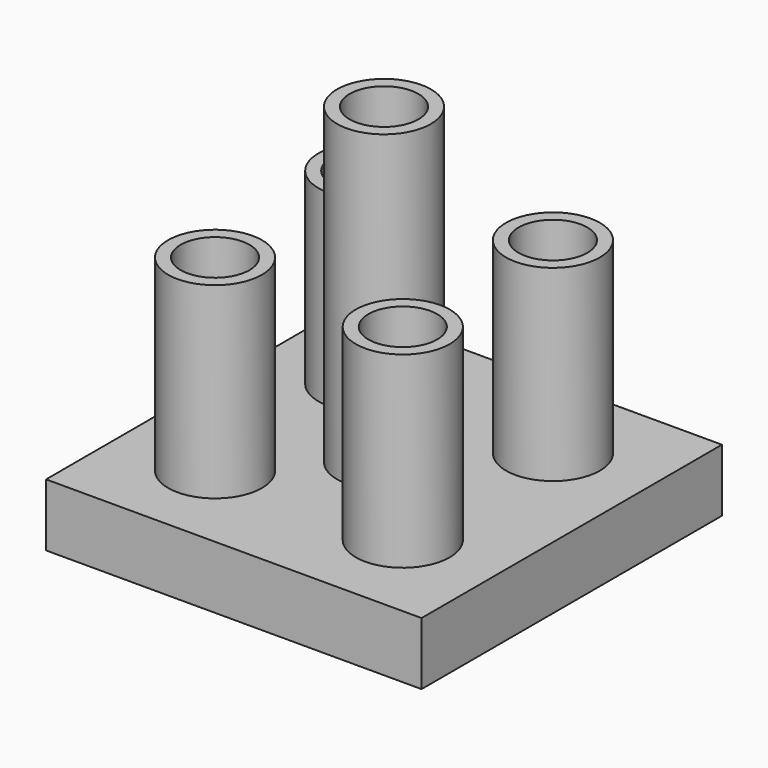
from build123d import *

# Parameters (mm, degrees)
F1_DEPTH    = 12.7
F2_R        = 9.525
F3_DEPTH    = 38.1
F4_T        = -2.54
F5_R        = 9.525
F6_DEPTH    = 63.5
F7_T        = 2.54
F7_T3_DEPTH = 12.7
F7_T5_DEPTH = 76.2
F7_T7_DEPTH = 76.2


# Not quite as in the source:
# - a shell that OpenCascade refuses in one call is made with other operations: the cavity is built on its own and cut out


with BuildPart() as f1:
    # F0 (on Top) → F1 (new body)
    with BuildSketch(Plane.XY):
        Polygon((-18.9360706136, 32.5840498031), (-57.0360706136, 32.5840498031), (-57.0360706136, -5.5159501969), (-57.0360706136, -43.6159501969), (-18.9360706136, -43.6159501969), (19.1639293864, -43.6159501969), (19.1639293864, -5.5159501969), (19.1639293864, 32.5840498031), align=None)
    extrude(amount=F1_DEPTH)

    # F2 (on face) → F3 (join)
    with BuildSketch(Plane.XY.offset(12.7)):
        with Locations((-37.9860706136, 13.5340498031)):
            Circle(F2_R)
        with Locations((0.1139293864, 13.5340498031)):
            Circle(F2_R)
        with Locations((-37.9860706136, -24.5659501969)):
            Circle(F2_R)
        with Locations((0.1139293864, -24.5659501969)):
            Circle(F2_R)
    extrude(amount=F3_DEPTH)

    # F4
    f4_openings = [f1.faces().sort_by_distance(p)[0] for p in [
        (0.113929, 13.53405, 50.8),
        (0.113929, -24.56595, 50.8),
        (-37.986071, -24.56595, 50.8),
        (-37.986071, 13.53405, 50.8),
    ]]
    offset(amount=F4_T, openings=f4_openings, kind=Kind.INTERSECTION)

    # F5 (on face) → F6 (join)
    with BuildSketch(Plane.XY.offset(12.7)):
        with Locations((-18.9360706136, -5.5159501969)):
            Circle(F5_R)
    extrude(amount=F6_DEPTH)

    # F7: shell of thickness 2.54, made by hand


with BuildPart() as f7_core1:
    # F7_t2: copy of F1
    add(f1.part)

    # the walls: a layer under each face that stays
    f7_faces = [f7_core1.faces().sort_by_distance(p)[0] for p in [
        (-18.9360706136, 30.0440498031, 6.35),
        (16.6239293864, -5.5159501969, 6.35),
        (-18.9360706136, -5.5159501969, 10.16),
        (-54.4960706136, -5.5159501969, 6.35),
        (-18.9360706136, -5.5159501969, 2.54),
        (-18.9360706136, -41.0759501969, 6.35),
        (-44.9710706136, 13.5340498031, 30.48),
        (-44.9710706136, -24.5659501969, 30.48),
        (-6.8710706136, 13.5340498031, 30.48),
        (-6.8710706136, -24.5659501969, 30.48),
        (-44.3360706136, 7.1840498031, 50.8),
        (-44.3360706136, -30.9159501969, 50.8),
        (-6.2360706136, 7.1840498031, 50.8),
        (-6.2360706136, -30.9159501969, 50.8),
        (-47.5110706136, 13.5340498031, 31.75),
        (-47.5110706136, -24.5659501969, 31.75),
        (-9.4110706136, 13.5340498031, 31.75),
        (-9.4110706136, -24.5659501969, 31.75),
        (-44.3360706136, -5.5159501969, 12.7),
        (-18.9360706136, 32.5840498031, 6.35),
        (-57.0360706136, -5.5159501969, 6.35),
        (19.1639293864, -5.5159501969, 6.35),
        (-18.9360706136, -43.6159501969, 6.35),
        (-28.4610706136, -5.5159501969, 44.45),
        (-18.9360706136, -5.5159501969, 0),
    ]]
    thicken(f7_faces, amount=-F7_T, mode=Mode.SUBTRACT)

    # F7_s4 → F7_t3 (cut)
    with BuildSketch(Plane.XY):
        Polygon((16.5985293864, 30.0186498031), (16.6239293864, 32.5840498031), (19.1639293864, 32.5840498031), (19.1639293864, 30.0440498031), align=None)
        Polygon((-54.4706706136, 30.0186498031), (-54.4960706136, 32.5840498031), (-57.0360706136, 32.5840498031), (-57.0360706136, 30.0440498031), align=None)
        Polygon((16.5985293864, -41.0505501969), (19.1639293864, -41.0759501969), (19.1639293864, -43.6159501969), (16.6239293864, -43.6159501969), align=None)
        Polygon((-54.4706706136, -41.0505501969), (-57.0360706136, -41.0759501969), (-57.0360706136, -43.6159501969), (-54.4960706136, -43.6159501969), align=None)
    extrude(amount=F7_T3_DEPTH, mode=Mode.SUBTRACT)

    # F7_s6 → F7_t5 (cut)
    with BuildSketch(Plane.YZ.offset(-57.0360706136)):
        Polygon((30.0186498031, 10.1346), (32.5840498031, 10.16), (32.5840498031, 12.7), (30.0440498031, 12.7), align=None)
        Polygon((30.0186498031, 2.5654), (32.5840498031, 2.54), (32.5840498031, 0), (30.0440498031, 0), align=None)
        Polygon((-41.0505501969, 10.1346), (-41.0759501969, 12.7), (-43.6159501969, 12.7), (-43.6159501969, 10.16), align=None)
        Polygon((-41.0505501969, 2.5654), (-41.0759501969, 0), (-43.6159501969, 0), (-43.6159501969, 2.54), align=None)
    extrude(amount=F7_T5_DEPTH, mode=Mode.SUBTRACT)

    # F7_s8 → F7_t7 (cut)
    with BuildSketch(Plane.XZ.offset(-32.5840498031)):
        Polygon((16.5985293864, 10.1346), (19.1639293864, 10.16), (19.1639293864, 12.7), (16.6239293864, 12.7), align=None)
        Polygon((16.5985293864, 2.5654), (19.1639293864, 2.54), (19.1639293864, 0), (16.6239293864, 0), align=None)
        Polygon((-54.4706706136, 10.1346), (-54.4960706136, 12.7), (-57.0360706136, 12.7), (-57.0360706136, 10.16), align=None)
        Polygon((-54.4706706136, 2.5654), (-57.0360706136, 2.54), (-57.0360706136, 0), (-54.4960706136, 0), align=None)
    extrude(amount=F7_T7_DEPTH, mode=Mode.SUBTRACT)

    # F7_s9 → F7_t10 (revolve, cut)
    with BuildSketch(Plane.XZ.offset(-13.5340498031)):
        Polygon((-28.4356706136, 12.7254), (-31.0010706136, 12.7), (-31.0010706136, 10.16), (-28.4610706136, 10.16), align=None)
    revolve(axis=Axis((-37.9860706136, 13.5340498031, 12.7), (0, 0, 1)), mode=Mode.SUBTRACT)

    # F7_s11 → F7_t12 (revolve, cut)
    with BuildSketch(Plane.XZ.offset(24.5659501969)):
        Polygon((-28.4356706136, 12.7254), (-31.0010706136, 12.7), (-31.0010706136, 10.16), (-28.4610706136, 10.16), align=None)
    revolve(axis=Axis((-37.9860706136, -24.5659501969, 12.7), (0, 0, 1)), mode=Mode.SUBTRACT)

    # F7_s13 → F7_t14 (revolve, cut)
    with BuildSketch(Plane.XZ.offset(-13.5340498031)):
        Polygon((9.6643293864, 12.7254), (7.0989293864, 12.7), (7.0989293864, 10.16), (9.6389293864, 10.16), align=None)
    revolve(axis=Axis((0.1139293864, 13.5340498031, 12.7), (0, 0, 1)), mode=Mode.SUBTRACT)

    # F7_s15 → F7_t16 (revolve, cut)
    with BuildSketch(Plane.XZ.offset(24.5659501969)):
        Polygon((9.6643293864, 12.7254), (7.0989293864, 12.7), (7.0989293864, 10.16), (9.6389293864, 10.16), align=None)
    revolve(axis=Axis((0.1139293864, -24.5659501969, 12.7), (0, 0, 1)), mode=Mode.SUBTRACT)

    # F7_s17 → F7_t18 (revolve, cut)
    with BuildSketch(Plane.XZ.offset(5.5159501969)):
        Polygon((-9.3856706136, 12.7254), (-9.4110706136, 10.16), (-11.9510706136, 10.16), (-11.9510706136, 12.7), align=None)
    revolve(axis=Axis((-18.9360706136, -5.5159501969, 12.7), (0, 0, 1)), mode=Mode.SUBTRACT)


with BuildPart() as f1_1:
    add(f1.part)

    # what is left inside the walls is the cavity
    f7_cavity = [f7_core1.part.solids().sort_by_distance(p)[0] for p in [
        (-25.895671, -5.51595, 55.033333),
    ]]
    add(f7_cavity, mode=Mode.SUBTRACT)


solid = f1_1.part
